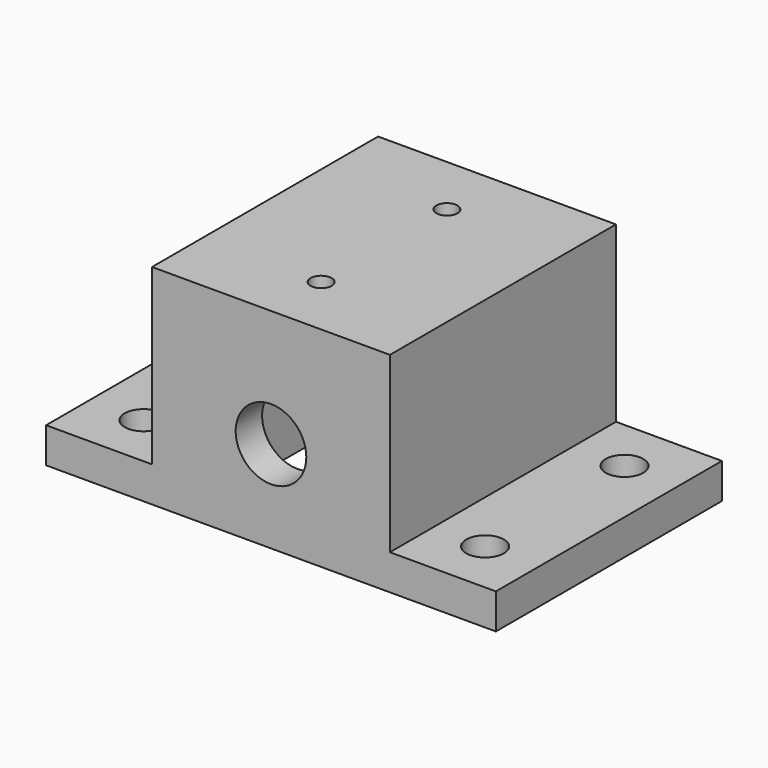
from build123d import *

# Parameters (mm, degrees)
F0_W      = 80.8736
F0_H      = 50.8
F1_DEPTH  = 37.592
F3_DEPTH  = 31.242
F4_W      = 30.85465
F4_H      = 38.89375
F5_DEPTH  = 31.242
F6_R      = 6.35
F7_DEPTH  = 25400
F8_DEPTH  = 31.242
F9_R      = 1.89865
F10_DEPTH = 25.4
F11_R     = 3.3782
F12_DEPTH = 25.4


# Not quite as in the source:
# - a feature names something its author has since deleted; it is built from what else it names


with BuildPart() as f1:
    # F0 (on Top) → F1 (new body)
    with BuildSketch(Plane.XY):
        Rectangle(F0_W, F0_H)
    extrude(amount=F1_DEPTH)

    # F2 (on face) → F3 (cut)
    with BuildSketch(Plane.XY.offset(37.592)):
        Polygon((40.4368, 25.4), (21.3868, 25.4), (21.3868, 19.05), (21.3868, -19.05), (21.3868, -25.4), (40.4368, -25.4), (40.4368, -19.05), (40.4368, 19.05), align=None)
    extrude(amount=-F3_DEPTH, mode=Mode.SUBTRACT)

    # F4 (on face) → F5 (cut)
    with BuildSketch(Plane(origin=(0, 0, 0), x_dir=(1, 0, 0), z_dir=(0, 0, -1))):
        Rectangle(F4_W, F4_H)
    extrude(amount=-F5_DEPTH, mode=Mode.SUBTRACT)

    # F6 (on face) → F7 (cut)
    with BuildSketch(Plane.XZ.offset(25.4)):
        with Locations((0, 16.51)):
            Circle(F6_R)
    extrude(amount=-F7_DEPTH, mode=Mode.SUBTRACT)

    # F2 (on face) → F8 (cut)
    with BuildSketch(Plane.XY.offset(37.592)):
        Polygon((-40.4368, 25.4), (-40.4368, 19.05), (-40.4368, -19.05), (-40.4368, -25.4), (-21.3868, -25.4), (-21.3868, -19.05), (-21.3868, 19.05), (-21.3868, 25.4), align=None)
    extrude(amount=-F8_DEPTH, mode=Mode.SUBTRACT)

    # F9 (on face) → F10 (cut)
    with BuildSketch(Plane.XY.offset(37.592)):
        with Locations((0, 14.14145)):
            Circle(F9_R)
        with Locations((0, -14.12875)):
            Circle(F9_R)
    extrude(amount=-F10_DEPTH, mode=Mode.SUBTRACT)

    # F11 (on face) → F12 (cut)
    with BuildSketch(Plane.XY.offset(6.35)):
        with Locations((-30.7086, 15.6718)):
            Circle(F11_R)
        with Locations((-30.7086, -15.6718)):
            Circle(F11_R)
        with Locations((30.7086, 15.6718)):
            Circle(F11_R)
        with Locations((30.7086, -15.6718)):
            Circle(F11_R)
    extrude(amount=-F12_DEPTH, mode=Mode.SUBTRACT)


solid = f1.part
